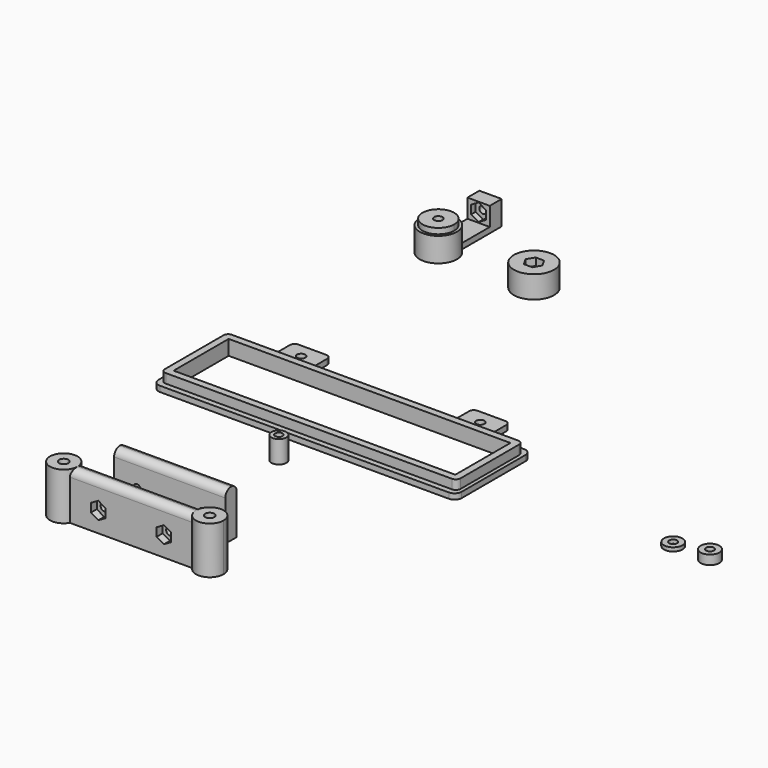
from build123d import *

# Parameters (mm, degrees)
F0_W           = 158.75
F0_H           = 44.45
F0_W_2         = 7
F0_H_2         = 3
F0_W_3         = 3
F0_H_3         = 7
F0_W_4         = 20
F0_H_4         = 15
F0_R           = 2.25
F0_W_5         = 137.25
F0_H_5         = 22.95
F1_DEPTH       = 3
F2_DEPTH       = 8
F3_R           = 2.54
F5_DEPTH       = 13
F6_DEPTH       = 9
F4_W           = 12
F4_H           = 8
F7_DEPTH       = 3
F8_START       = 5
F8_DEPTH       = 11
F9_DEPTH       = 13
F10_R          = 2
F11_DEPTH      = 25.4
F12_DEPTH      = 3
F12_DEPTH_BACK = 3
F13_R          = 10.795
F13_R_2        = 2.25
F14_DEPTH      = 12
F15_START      = 8
F15_DEPTH      = 17.4
F16_START      = 2
F16_DEPTH      = 23.4
F17_R          = 4
F17_R_2        = 2
F18_DEPTH      = 12
F19_R          = 2.5
F20_DEPTH      = 25.4
F21_R          = 3.80999
F22_R          = 2
F23_DEPTH      = 4
F24_DEPTH      = 25.4
F25_W          = 59.6999956
F25_H          = 7.62
F26_DEPTH      = 25.4
F27_R          = 3.80999
F28_R          = 2
F29_DEPTH      = 25.4
F30_R          = 5
F30_R_2        = 2.125
F31_DEPTH      = 2
F32_DEPTH      = 5


# Not quite as in the source:
# - a fillet or chamfer is up to 0.001 mm smaller than in the source, because OpenCascade refuses the exact size


with BuildPart() as f1:
    # F0 (on Top) → F1 (new body)
    with BuildSketch(Plane.XY):
        with BuildLine():
            Line((-77.565, -25.225), (77.565, -25.225))
            ThreePointArc((77.565, -25.225), (80.2590768363, -24.1090768363), (81.375, -21.415))
            Line((81.375, -21.415), (81.375, 21.415))
            ThreePointArc((81.375, 21.415), (80.2590768363, 24.1090768363), (77.565, 25.225))
            Line((77.565, 25.225), (58.1, 25.225))
            Line((58.1, 25.225), (38.1, 25.225))
            Line((38.1, 25.225), (-38.1, 25.225))
            Line((-38.1, 25.225), (-58.1, 25.225))
            Line((-58.1, 25.225), (-77.565, 25.225))
            ThreePointArc((-77.565, 25.225), (-80.2590768363, 24.1090768363), (-81.375, 21.415))
            Line((-81.375, 21.415), (-81.375, -21.415))
            ThreePointArc((-81.375, -21.415), (-80.2590768363, -24.1090768363), (-77.565, -25.225))
        make_face()
        Rectangle(F0_W, F0_H, mode=Mode.SUBTRACT)
        Rectangle(F0_W, F0_H)
        Polygon((-78.625, 18.475), (-78.625, 21.475), (-75.625, 21.475), (-68.625, 21.475), (68.625, 21.475), (75.625, 21.475), (78.625, 21.475), (78.625, 18.475), (78.625, 11.475), (75.625, 11.475), (75.625, -11.475), (78.625, -11.475), (78.625, -18.475), (78.625, -21.475), (75.625, -21.475), (68.625, -21.475), (-68.625, -21.475), (-75.625, -21.475), (-78.625, -21.475), (-78.625, -18.475), (-78.625, -11.475), (-78.625, 11.475), align=None, mode=Mode.SUBTRACT)
        with Locations((-72.125, 19.975)):
            Rectangle(F0_W_2, F0_H_2)
        with Locations((-77.125, 19.975)):
            Rectangle(F0_W_3, F0_H_2)
        with Locations((-77.125, 14.975)):
            Rectangle(F0_W_3, F0_H_3)
        with Locations((-77.125, -14.975)):
            Rectangle(F0_W_3, F0_H_3)
        with Locations((-77.125, -19.975)):
            Rectangle(F0_W_3, F0_H_2)
        with Locations((-72.125, -19.975)):
            Rectangle(F0_W_2, F0_H_2)
        with Locations((72.125, 19.975)):
            Rectangle(F0_W_2, F0_H_2)
        with Locations((77.125, 19.975)):
            Rectangle(F0_W_3, F0_H_2)
        with Locations((77.125, 14.975)):
            Rectangle(F0_W_3, F0_H_3)
        with Locations((77.125, -14.975)):
            Rectangle(F0_W_3, F0_H_3)
        with Locations((72.125, -19.975)):
            Rectangle(F0_W_2, F0_H_2)
        with Locations((77.125, -19.975)):
            Rectangle(F0_W_3, F0_H_2)
        with Locations((-48.1, 32.725)):
            Rectangle(F0_W_4, F0_H_4)
        with Locations((-48.1, 32.725)):
            Circle(F0_R, mode=Mode.SUBTRACT)
        with Locations((48.1, 32.725)):
            Rectangle(F0_W_4, F0_H_4)
        with Locations((48.1, 32.725)):
            Circle(F0_R, mode=Mode.SUBTRACT)
        with Locations((0, 19.975)):
            Rectangle(F0_W_5, F0_H_2)
        with Locations((-77.125, 0)):
            Rectangle(F0_W_3, F0_H_5)
        with Locations((0, -19.975)):
            Rectangle(F0_W_5, F0_H_2)
    extrude(amount=F1_DEPTH)

    # F0 (on Top) → F2 (join)
    with BuildSketch(Plane.XY):
        Rectangle(F0_W, F0_H)
        Polygon((-78.625, 18.475), (-78.625, 21.475), (-75.625, 21.475), (-68.625, 21.475), (68.625, 21.475), (75.625, 21.475), (78.625, 21.475), (78.625, 18.475), (78.625, 11.475), (75.625, 11.475), (75.625, -11.475), (78.625, -11.475), (78.625, -18.475), (78.625, -21.475), (75.625, -21.475), (68.625, -21.475), (-68.625, -21.475), (-75.625, -21.475), (-78.625, -21.475), (-78.625, -18.475), (-78.625, -11.475), (-78.625, 11.475), align=None, mode=Mode.SUBTRACT)
        with Locations((0, 19.975)):
            Rectangle(F0_W_5, F0_H_2)
        with Locations((0, -19.975)):
            Rectangle(F0_W_5, F0_H_2)
        with Locations((-77.125, 0)):
            Rectangle(F0_W_3, F0_H_5)
        with Locations((72.125, 19.975)):
            Rectangle(F0_W_2, F0_H_2)
        with Locations((77.125, 14.975)):
            Rectangle(F0_W_3, F0_H_3)
        with Locations((77.125, -14.975)):
            Rectangle(F0_W_3, F0_H_3)
        with Locations((72.125, -19.975)):
            Rectangle(F0_W_2, F0_H_2)
        with Locations((-72.125, 19.975)):
            Rectangle(F0_W_2, F0_H_2)
        with Locations((-77.125, 14.975)):
            Rectangle(F0_W_3, F0_H_3)
        with Locations((-77.125, -14.975)):
            Rectangle(F0_W_3, F0_H_3)
        with Locations((-72.125, -19.975)):
            Rectangle(F0_W_2, F0_H_2)
        with Locations((77.125, 19.975)):
            Rectangle(F0_W_3, F0_H_2)
        with Locations((77.125, -19.975)):
            Rectangle(F0_W_3, F0_H_2)
        with Locations((-77.125, 19.975)):
            Rectangle(F0_W_3, F0_H_2)
        with Locations((-77.125, -19.975)):
            Rectangle(F0_W_3, F0_H_2)
    extrude(amount=F2_DEPTH)

    # F3
    f3_edges = [f1.edges().sort_by_distance(p)[0] for p in [
        (58.1, 40.225, 1.5),
        (38.1, 40.225, 1.5),
        (-38.1, 40.225, 1.5),
        (-58.1, 40.225, 1.5),
        (-79.375, 22.225, 5.5),
        (-79.375, -22.225, 5.5),
        (79.375, 22.225, 5.5),
        (79.375, -22.225, 5.5),
    ]]
    fillet(f3_edges, radius=F3_R)


with BuildPart() as f5:
    # F4 (on Top) → F5 (new body)
    with BuildSketch(Plane.XY):
        with BuildLine():
            ThreePointArc((-57.1067942702, 146.6848796847), (-57.7566350361, 149.9444808873), (-59.6067942702, 152.7056769741))
            Line((-59.6067942702, 152.7056769741), (-59.6067942702, 146.6848796847))
            Line((-59.6067942702, 146.6848796847), (-61.6067942702, 146.6848796847))
            Line((-61.6067942702, 146.6848796847), (-61.6067942702, 144.375478608))
            Line((-61.6067942702, 144.375478608), (-65.6067942702, 142.0660775312))
            Line((-65.6067942702, 142.0660775312), (-69.6067942702, 144.375478608))
            Line((-69.6067942702, 144.375478608), (-69.6067942702, 146.6848796847))
            Line((-69.6067942702, 146.6848796847), (-71.6067942702, 146.6848796847))
            Line((-71.6067942702, 146.6848796847), (-71.6067942702, 152.7056769741))
            ThreePointArc((-71.6067942702, 152.7056769741), (-68.8663954728, 138.8347204507), (-57.1067942702, 146.6848796847))
        make_face()
        with BuildLine():
            ThreePointArc((-71.6067942702, 154.6848796847), (-70.0789302252, 137.7406077747), (-55.6067942702, 146.6848796847))
            ThreePointArc((-55.6067942702, 146.6848796847), (-56.6625223602, 151.1570156397), (-59.6067942702, 154.6848796847))
            Line((-59.6067942702, 154.6848796847), (-59.6067942702, 152.7056769741))
            ThreePointArc((-59.6067942702, 152.7056769741), (-57.7566350361, 149.9444808873), (-57.1067942702, 146.6848796847))
            ThreePointArc((-57.1067942702, 146.6848796847), (-68.8663954728, 138.8347204507), (-71.6067942702, 152.7056769741))
            Line((-71.6067942702, 152.7056769741), (-71.6067942702, 154.6848796847))
        make_face()
        with BuildLine():
            Line((-59.6067942702, 146.6848796847), (-59.6067942702, 152.7056769741))
            ThreePointArc((-59.6067942702, 152.7056769741), (-65.6067942702, 155.1848796847), (-71.6067942702, 152.7056769741))
            Line((-71.6067942702, 152.7056769741), (-71.6067942702, 146.6848796847))
            Line((-71.6067942702, 146.6848796847), (-69.6067942702, 146.6848796847))
            Line((-69.6067942702, 146.6848796847), (-69.6067942702, 148.9942807615))
            Line((-69.6067942702, 148.9942807615), (-65.6067942702, 151.3036818383))
            Line((-65.6067942702, 151.3036818383), (-61.6067942702, 148.9942807615))
            Line((-61.6067942702, 148.9942807615), (-61.6067942702, 146.6848796847))
            Line((-61.6067942702, 146.6848796847), (-59.6067942702, 146.6848796847))
        make_face()
        with BuildLine():
            Line((-59.6067942702, 152.7056769741), (-59.6067942702, 154.6848796847))
            ThreePointArc((-59.6067942702, 154.6848796847), (-65.6067942702, 156.6848796847), (-71.6067942702, 154.6848796847))
            Line((-71.6067942702, 154.6848796847), (-71.6067942702, 152.7056769741))
            ThreePointArc((-71.6067942702, 152.7056769741), (-65.6067942702, 155.1848796847), (-59.6067942702, 152.7056769741))
        make_face()
        with BuildLine():
            Line((-63.3567942702, 146.6848796847), (-61.6067942702, 146.6848796847))
            Line((-61.6067942702, 146.6848796847), (-61.6067942702, 148.9942807615))
            Line((-61.6067942702, 148.9942807615), (-65.6067942702, 151.3036818383))
            Line((-65.6067942702, 151.3036818383), (-69.6067942702, 148.9942807615))
            Line((-69.6067942702, 148.9942807615), (-69.6067942702, 146.6848796847))
            Line((-69.6067942702, 146.6848796847), (-67.8567942702, 146.6848796847))
            ThreePointArc((-67.8567942702, 146.6848796847), (-65.6067942702, 148.9348796847), (-63.3567942702, 146.6848796847))
        make_face()
        with BuildLine():
            Line((-61.6067942702, 144.375478608), (-61.6067942702, 146.6848796847))
            Line((-61.6067942702, 146.6848796847), (-63.3567942702, 146.6848796847))
            ThreePointArc((-63.3567942702, 146.6848796847), (-65.6067942702, 144.4348796847), (-67.8567942702, 146.6848796847))
            Line((-67.8567942702, 146.6848796847), (-69.6067942702, 146.6848796847))
            Line((-69.6067942702, 146.6848796847), (-69.6067942702, 144.375478608))
            Line((-69.6067942702, 144.375478608), (-65.6067942702, 142.0660775312))
            Line((-65.6067942702, 142.0660775312), (-61.6067942702, 144.375478608))
        make_face()
    extrude(amount=F5_DEPTH)

    # F4 (on Top) → F6 (cut)
    with BuildSketch(Plane.XY):
        with BuildLine():
            Line((-61.6067942702, 144.375478608), (-61.6067942702, 146.6848796847))
            Line((-61.6067942702, 146.6848796847), (-63.3567942702, 146.6848796847))
            ThreePointArc((-63.3567942702, 146.6848796847), (-65.6067942702, 144.4348796847), (-67.8567942702, 146.6848796847))
            Line((-67.8567942702, 146.6848796847), (-69.6067942702, 146.6848796847))
            Line((-69.6067942702, 146.6848796847), (-69.6067942702, 144.375478608))
            Line((-69.6067942702, 144.375478608), (-65.6067942702, 142.0660775312))
            Line((-65.6067942702, 142.0660775312), (-61.6067942702, 144.375478608))
        make_face()
        with BuildLine():
            Line((-63.3567942702, 146.6848796847), (-61.6067942702, 146.6848796847))
            Line((-61.6067942702, 146.6848796847), (-61.6067942702, 148.9942807615))
            Line((-61.6067942702, 148.9942807615), (-65.6067942702, 151.3036818383))
            Line((-65.6067942702, 151.3036818383), (-69.6067942702, 148.9942807615))
            Line((-69.6067942702, 148.9942807615), (-69.6067942702, 146.6848796847))
            Line((-69.6067942702, 146.6848796847), (-67.8567942702, 146.6848796847))
            ThreePointArc((-67.8567942702, 146.6848796847), (-65.6067942702, 148.9348796847), (-63.3567942702, 146.6848796847))
        make_face()
    extrude(amount=F6_DEPTH, mode=Mode.SUBTRACT)

    # F4 (on Top) → F7 (join)
    with BuildSketch(Plane.XY):
        with BuildLine():
            Line((-59.6067942702, 152.7056769741), (-59.6067942702, 154.6848796847))
            ThreePointArc((-59.6067942702, 154.6848796847), (-65.6067942702, 156.6848796847), (-71.6067942702, 154.6848796847))
            Line((-71.6067942702, 154.6848796847), (-71.6067942702, 152.7056769741))
            ThreePointArc((-71.6067942702, 152.7056769741), (-65.6067942702, 155.1848796847), (-59.6067942702, 152.7056769741))
        make_face()
        with BuildLine():
            ThreePointArc((-71.6067942702, 154.6848796847), (-65.6067942702, 156.6848796847), (-59.6067942702, 154.6848796847))
            Line((-59.6067942702, 154.6848796847), (-59.6067942702, 173.6848796847))
            Line((-59.6067942702, 173.6848796847), (-71.6067942702, 173.6848796847))
            Line((-71.6067942702, 173.6848796847), (-71.6067942702, 154.6848796847))
        make_face()
        with Locations((-65.6067942702, 177.6848796847)):
            Rectangle(F4_W, F4_H)
    extrude(amount=F7_DEPTH)

    # F4 (on Top) → F8 (join)
    with BuildSketch(Plane.XY.offset(F8_START)):
        with BuildLine():
            ThreePointArc((-57.1067942702, 146.6848796847), (-57.7566350361, 149.9444808873), (-59.6067942702, 152.7056769741))
            Line((-59.6067942702, 152.7056769741), (-59.6067942702, 146.6848796847))
            Line((-59.6067942702, 146.6848796847), (-61.6067942702, 146.6848796847))
            Line((-61.6067942702, 146.6848796847), (-61.6067942702, 144.375478608))
            Line((-61.6067942702, 144.375478608), (-65.6067942702, 142.0660775312))
            Line((-65.6067942702, 142.0660775312), (-69.6067942702, 144.375478608))
            Line((-69.6067942702, 144.375478608), (-69.6067942702, 146.6848796847))
            Line((-69.6067942702, 146.6848796847), (-71.6067942702, 146.6848796847))
            Line((-71.6067942702, 146.6848796847), (-71.6067942702, 152.7056769741))
            ThreePointArc((-71.6067942702, 152.7056769741), (-68.8663954728, 138.8347204507), (-57.1067942702, 146.6848796847))
        make_face()
        with BuildLine():
            Line((-59.6067942702, 146.6848796847), (-59.6067942702, 152.7056769741))
            ThreePointArc((-59.6067942702, 152.7056769741), (-65.6067942702, 155.1848796847), (-71.6067942702, 152.7056769741))
            Line((-71.6067942702, 152.7056769741), (-71.6067942702, 146.6848796847))
            Line((-71.6067942702, 146.6848796847), (-69.6067942702, 146.6848796847))
            Line((-69.6067942702, 146.6848796847), (-69.6067942702, 148.9942807615))
            Line((-69.6067942702, 148.9942807615), (-65.6067942702, 151.3036818383))
            Line((-65.6067942702, 151.3036818383), (-61.6067942702, 148.9942807615))
            Line((-61.6067942702, 148.9942807615), (-61.6067942702, 146.6848796847))
            Line((-61.6067942702, 146.6848796847), (-59.6067942702, 146.6848796847))
        make_face()
        with BuildLine():
            Line((-63.3567942702, 146.6848796847), (-61.6067942702, 146.6848796847))
            Line((-61.6067942702, 146.6848796847), (-61.6067942702, 148.9942807615))
            Line((-61.6067942702, 148.9942807615), (-65.6067942702, 151.3036818383))
            Line((-65.6067942702, 151.3036818383), (-69.6067942702, 148.9942807615))
            Line((-69.6067942702, 148.9942807615), (-69.6067942702, 146.6848796847))
            Line((-69.6067942702, 146.6848796847), (-67.8567942702, 146.6848796847))
            ThreePointArc((-67.8567942702, 146.6848796847), (-65.6067942702, 148.9348796847), (-63.3567942702, 146.6848796847))
        make_face()
        with BuildLine():
            Line((-61.6067942702, 144.375478608), (-61.6067942702, 146.6848796847))
            Line((-61.6067942702, 146.6848796847), (-63.3567942702, 146.6848796847))
            ThreePointArc((-63.3567942702, 146.6848796847), (-65.6067942702, 144.4348796847), (-67.8567942702, 146.6848796847))
            Line((-67.8567942702, 146.6848796847), (-69.6067942702, 146.6848796847))
            Line((-69.6067942702, 146.6848796847), (-69.6067942702, 144.375478608))
            Line((-69.6067942702, 144.375478608), (-65.6067942702, 142.0660775312))
            Line((-65.6067942702, 142.0660775312), (-61.6067942702, 144.375478608))
        make_face()
    extrude(amount=F8_DEPTH)

    # F4 (on Top) → F9 (join)
    with BuildSketch(Plane.XY):
        with Locations((-65.6067942702, 177.6848796847)):
            Rectangle(F4_W, F4_H)
    extrude(amount=F9_DEPTH)

    # F10 (on face) → F11 (cut)
    with BuildSketch(Plane.XZ.offset(-173.6848796847)):
        with Locations((-65.6067942702, 8)):
            Circle(F10_R)
    extrude(amount=-F11_DEPTH, mode=Mode.SUBTRACT)

    # F10 (on face) → F12 (cut, two sides)
    with BuildSketch(Plane.XZ.offset(-173.6848796847)) as f12_sk:
        Polygon((-65.6067942702, 3.3811978465), (-61.6067942702, 5.6905989232), (-61.6067942702, 10.3094010768), (-65.6067942702, 12.6188021535), (-69.6067942702, 10.3094010768), (-69.6067942702, 5.6905989232), align=None)
        with Locations((-65.6067942702, 8)):
            Circle(F10_R, mode=Mode.SUBTRACT)
    extrude(amount=-F12_DEPTH, mode=Mode.SUBTRACT)
    extrude(f12_sk.sketch, amount=F12_DEPTH_BACK, mode=Mode.SUBTRACT)


with BuildPart() as f14:
    # F13 (on Top) → F14 (new body)
    with BuildSketch(Plane.XY):
        with Locations((-14.2757417634, 146.6848796847)):
            Circle(F13_R)
        Polygon((-11.956968477, 150.5789936763), (-9.7439534783, 146.6238201089), (-12.0627267646, 142.7297061173), (-16.5945150498, 142.7907656931), (-18.8075300486, 146.7459392606), (-16.4887567622, 150.6400532522), align=None, mode=Mode.SUBTRACT)
        Polygon((-12.0627267646, 142.7297061173), (-9.7439534783, 146.6238201089), (-11.956968477, 150.5789936763), (-16.4887567622, 150.6400532522), (-18.8075300486, 146.7459392606), (-16.5945150498, 142.7907656931), align=None)
        with Locations((-14.2757417634, 146.6848796847)):
            Circle(F13_R_2, mode=Mode.SUBTRACT)
        with Locations((-14.2757417634, 146.6848796847)):
            Circle(F13_R_2)
    extrude(amount=F14_DEPTH)

    # F13 (on Top) → F15 (cut)
    with BuildSketch(Plane.XY.offset(F15_START)):
        Polygon((-12.0627267646, 142.7297061173), (-9.7439534783, 146.6238201089), (-11.956968477, 150.5789936763), (-16.4887567622, 150.6400532522), (-18.8075300486, 146.7459392606), (-16.5945150498, 142.7907656931), align=None)
        with Locations((-14.2757417634, 146.6848796847)):
            Circle(F13_R_2, mode=Mode.SUBTRACT)
        with Locations((-14.2757417634, 146.6848796847)):
            Circle(F13_R_2)
    extrude(amount=F15_DEPTH, mode=Mode.SUBTRACT)

    # F13 (on Top) → F16 (cut)
    with BuildSketch(Plane.XY.offset(F16_START)):
        with Locations((-14.2757417634, 146.6848796847)):
            Circle(F13_R_2)
    extrude(amount=F16_DEPTH, mode=Mode.SUBTRACT)


with BuildPart() as f18:
    # F17 (on Top) → F18 (new body)
    with BuildSketch(Plane.XY):
        with Locations((0, -42.3521701418)):
            Circle(F17_R)
        with Locations((0, -42.3521701418)):
            Circle(F17_R_2, mode=Mode.SUBTRACT)
    extrude(amount=F18_DEPTH)


with BuildPart() as f20:
    # F19 (on Top) → F20 (new body)
    with BuildSketch(Plane.XY):
        with BuildLine():
            ThreePointArc((32.8499978, -133.9236030521), (31.7946888935, -137.7336030521), (32.8499978, -141.5436030521))
            Line((32.8499978, -141.5436030521), (32.8499978, -137.7336030521))
            Line((32.8499978, -137.7336030521), (32.8499978, -133.9236030521))
        make_face()
        with BuildLine():
            Line((-32.8499978, -141.5436030521), (32.8499978, -141.5436030521))
            ThreePointArc((32.8499978, -141.5436030521), (31.7946888935, -137.7336030521), (32.8499978, -133.9236030521))
            Line((32.8499978, -133.9236030521), (-32.8499978, -133.9236030521))
            ThreePointArc((-32.8499978, -133.9236030521), (-32.0633910588, -135.7568774206), (-31.7946888935, -137.7336030521))
            ThreePointArc((-31.7946888935, -137.7336030521), (-32.0633910588, -139.7103286835), (-32.8499978, -141.5436030521))
        make_face()
        with BuildLine():
            Line((32.8499978, -137.7336030521), (32.8499978, -141.5436030521))
            ThreePointArc((32.8499978, -141.5436030521), (41.1767234314, -144.8702097932), (46.6053067065, -137.7336030521))
            ThreePointArc((46.6053067065, -137.7336030521), (41.1767234314, -130.5969963109), (32.8499978, -133.9236030521))
            Line((32.8499978, -133.9236030521), (32.8499978, -137.7336030521))
        make_face()
        with BuildLine():
            ThreePointArc((41.6999978, -137.7336030521), (39.1999978, -140.2336030521), (36.6999978, -137.7336030521))
            ThreePointArc((36.6999978, -137.7336030521), (39.1999978, -135.2336030521), (41.6999978, -137.7336030521))
        make_face(mode=Mode.SUBTRACT)
        with BuildLine():
            ThreePointArc((-32.8499978, -133.9236030521), (-46.6053067065, -137.7336030521), (-32.8499978, -141.5436030521))
            Line((-32.8499978, -141.5436030521), (-32.8499978, -137.7336030521))
            Line((-32.8499978, -137.7336030521), (-32.8499978, -133.9236030521))
        make_face()
        with Locations((-39.1999978, -137.7336030521)):
            Circle(F19_R, mode=Mode.SUBTRACT)
        with BuildLine():
            Line((-32.8499978, -137.7336030521), (-32.8499978, -141.5436030521))
            ThreePointArc((-32.8499978, -141.5436030521), (-32.0633910588, -139.7103286835), (-31.7946888935, -137.7336030521))
            ThreePointArc((-31.7946888935, -137.7336030521), (-32.0633910588, -135.7568774206), (-32.8499978, -133.9236030521))
            Line((-32.8499978, -133.9236030521), (-32.8499978, -137.7336030521))
        make_face()
    extrude(amount=F20_DEPTH)

    # F21 (radius 3.81 in the source; OpenCascade refuses exactly that, so slightly less here)
    f21_edges = [f20.edges().sort_by_distance(p)[0] for p in [
        (0, -133.923603, 25.4),
        (0, -141.543603, 25.4),
    ]]
    fillet(f21_edges, radius=F21_R)

    # F22 (on face) → F23 (cut)
    with BuildSketch(Plane.XZ.offset(141.5436030521)):
        Polygon((-17.6099978, 6.1761978465), (-13.6099978, 8.4855989232), (-13.6099978, 13.1044010768), (-17.6099978, 15.4138021535), (-21.6099978, 13.1044010768), (-21.6099978, 8.4855989232), align=None)
        with Locations((-17.6099978, 10.795)):
            Circle(F22_R, mode=Mode.SUBTRACT)
        Polygon((17.6099978, 6.2856743966), (21.5151883265, 8.5403371983), (21.5151883265, 13.0496628017), (17.6099978, 15.3043256034), (13.7048072735, 13.0496628017), (13.7048072735, 8.5403371983), align=None)
        with Locations((17.6099978, 10.795)):
            Circle(F22_R, mode=Mode.SUBTRACT)
    extrude(amount=-F23_DEPTH, mode=Mode.SUBTRACT)

    # F22 (on face) → F24 (cut)
    with BuildSketch(Plane.XZ.offset(141.5436030521)):
        with Locations((-17.6099978, 10.795)):
            Circle(F22_R)
        with Locations((17.6099978, 10.795)):
            Circle(F22_R)
    extrude(amount=-F24_DEPTH, mode=Mode.SUBTRACT)


with BuildPart() as f26:
    # F25 (on Top) → F26 (new body)
    with BuildSketch(Plane.XY):
        with Locations((0, -111.8036122029)):
            Rectangle(F25_W, F25_H)
    extrude(amount=F26_DEPTH)

    # F27 (radius 3.81 in the source; OpenCascade refuses exactly that, so slightly less here)
    f27_edges = [f26.edges().sort_by_distance(p)[0] for p in [
        (0, -115.613612, 25.4),
        (0, -107.993612, 25.4),
    ]]
    fillet(f27_edges, radius=F27_R)

    # F28 (on face) → F29 (cut)
    with BuildSketch(Plane.XZ.offset(115.6136122029)):
        with Locations((-17.6099978, 10.795)):
            Circle(F28_R)
        with Locations((17.6099978, 10.795)):
            Circle(F28_R)
    extrude(amount=-F29_DEPTH, mode=Mode.SUBTRACT)


with BuildPart() as f31:
    # F30 (on Top) → F31 (new body)
    with BuildSketch(Plane.XY):
        with Locations((177.8, 0)):
            Circle(F30_R)
        with Locations((177.8, 0)):
            Circle(F30_R_2, mode=Mode.SUBTRACT)
    extrude(amount=F31_DEPTH)


with BuildPart() as f32:
    # F30 (on Top) → F32 (new body)
    with BuildSketch(Plane.XY):
        with Locations((197.5803822279, 0)):
            Circle(F30_R)
        with Locations((197.5803822279, 0)):
            Circle(F30_R_2, mode=Mode.SUBTRACT)
    extrude(amount=F32_DEPTH)


solid = Compound([f1.part, f5.part, f14.part, f18.part, f20.part, f26.part, f31.part, f32.part])
